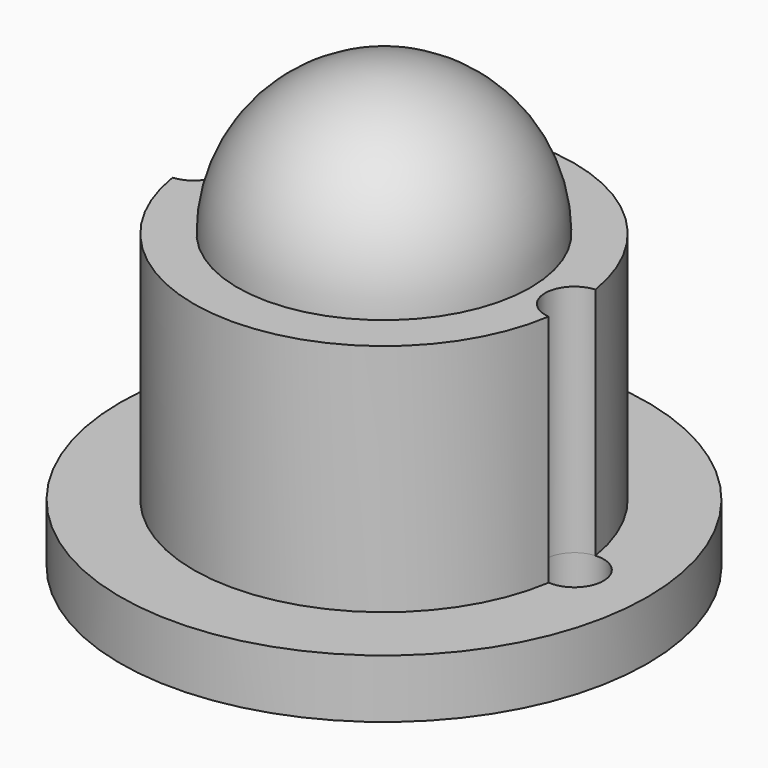
from build123d import *
from build123d import SkipClean  # not in build123d's __all__

# Parameters (mm, degrees)
F2_R     = 9
F2_R_2   = 1
F3_DEPTH = 2
F6_R     = 5
F7_DEPTH = 8


with BuildPart() as f3:
    # F2 (on Top) → F3 (new body)
    with BuildSketch(Plane.XY):
        Circle(F2_R)
        with Locations((-6.5, 0)):
            Circle(F2_R_2, mode=Mode.SUBTRACT)
        with Locations((6.5, 0)):
            Circle(F2_R_2, mode=Mode.SUBTRACT)
    extrude(amount=F3_DEPTH)



with BuildPart() as f5:
    # F4 (on Front) → F5 (revolve)
    with BuildSketch(Plane.XZ):
        with BuildLine():
            Line((0, 5), (0, 15))
            ThreePointArc((0, 15), (-5, 10), (0, 5))
        make_face()
    revolve(axis=Axis((0, 0, 8.2231094215), (0, 0, 1)))


with BuildPart() as f3_1:
    add(f3.part, clean=False)

    with SkipClean():  # cleaning this boolean's faces spoils the solid; the shape is the same uncleaned
        add(f5.part)  # F7 merges F5
    # F6 (on face) → F7 (join)
    with BuildSketch(Plane.XY.offset(2)):
        with BuildLine():
            ThreePointArc((6.4230769231, -0.9970370305), (5.5, 0), (6.4230769231, 0.9970370305))
            ThreePointArc((6.4230769231, 0.9970370305), (0, 6.5), (-6.4230769231, 0.9970370305))
            ThreePointArc((-6.4230769231, 0.9970370305), (-5.7662006143, 0.6793662205), (-5.5, 0))
            ThreePointArc((-5.5, 0), (-5.7662006143, -0.6793662205), (-6.4230769231, -0.9970370305))
            ThreePointArc((-6.4230769231, -0.9970370305), (0, -6.5), (6.4230769231, -0.9970370305))
        make_face()
        Circle(F6_R, mode=Mode.SUBTRACT)
    with SkipClean():  # cleaning this boolean's faces spoils the solid; the shape is the same uncleaned
        extrude(amount=F7_DEPTH)


solid = f3_1.part
